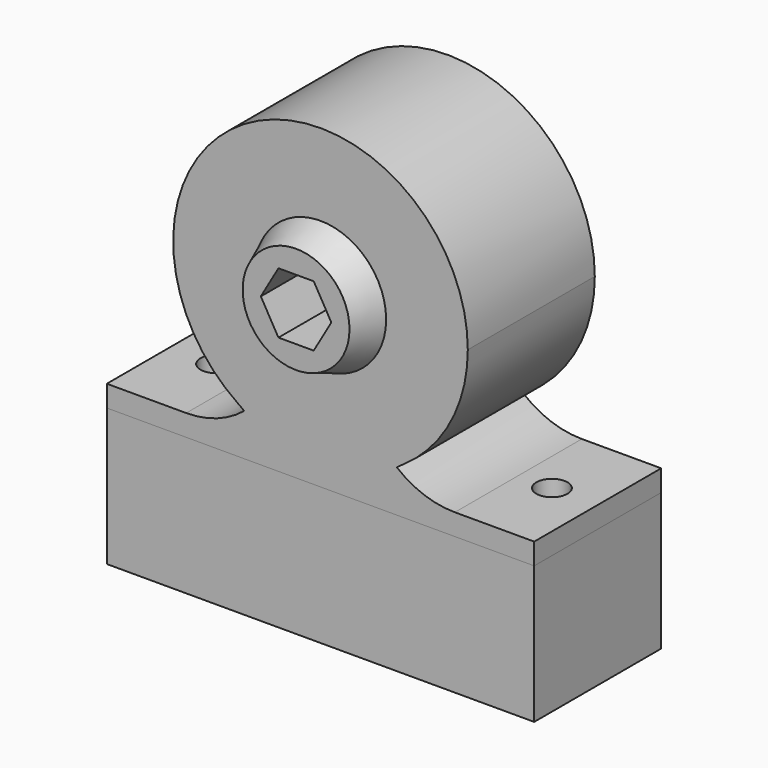
from build123d import *

# Parameters (mm, degrees)
F0_R         = 10.75
F1_DEPTH     = 26
F2_W         = 14
F2_H         = 26
F3_DEPTH     = 2
F4_T1_DEPTH  = 26
F4_T6_DEPTH  = 26
F4_T11_DEPTH = 26
F5_DEPTH     = 31
F6_SIZE2     = 5
F6_SIZE      = 2
F7_D         = 5.1054
F8_DEPTH     = 22.5


# Not quite as in the source:
# - a fillet or chamfer that OpenCascade refuses, or shapes differently, is made with other operations: its cross-section is extruded or revolved along the edge and cut away or added


with BuildPart() as f1:
    # F0 (on Front) → F1 (new body)
    with BuildSketch(Plane.XZ):
        with BuildLine():
            ThreePointArc((4.14e-08, -24.125), (17.0589511108, -17.0589510815), (24.125, 0))
            ThreePointArc((24.125, 0), (-17.0589511108, 17.0589510815), (4.14e-08, -24.125))
        make_face()
        Circle(F0_R, mode=Mode.SUBTRACT)
    extrude(amount=F1_DEPTH)



with BuildPart() as f1b:
    # F0 (on Front) → F1, piece 2 (new body)
    with BuildSketch(Plane.XZ):
        Polygon((35, -24.125), (4.14e-08, -24.125), (-35, -24.125), (-35, -27.625), (35, -27.625), align=None)
    extrude(amount=F1_DEPTH)


with BuildPart() as f1_1:
    add(f1.part)

    add(f1b.part)  # F3 merges F1b
    # F2 (on face) → F3 (join)
    with BuildSketch(Plane.XY.offset(-24.125)):
        with Locations((0, -13)):
            Rectangle(F2_W, F2_H)
    extrude(amount=F3_DEPTH)

    # F4: fillet of radius 15 on 4 edges, made by hand

    # F4_s2 → F4_t1 (join)
    with BuildSketch(Plane.XZ):
        with BuildLine():
            ThreePointArc((-22, -24.125), (-11.3933982822, -19.7316017178), (-7, -9.125))
            Line((-7, -9.125), (-7, -24.125))
            Line((-7, -24.125), (-22, -24.125))
        make_face()
        with BuildLine():
            ThreePointArc((22, -24.125), (11.3933982822, -19.7316017178), (7, -9.125))
            Line((7, -9.125), (7, -24.125))
            Line((7, -24.125), (22, -24.125))
        make_face()
    extrude(amount=F4_T1_DEPTH)


with BuildPart() as f4_tool4:
    # F4_s5 → F4_t6 (new body)
    with BuildSketch(Plane.XZ.offset(26)):
        with BuildLine():
            ThreePointArc((7, -32.3537575098), (8.7425950525, -25.3365490863), (13.5654952077, -19.9497610204))
            ThreePointArc((13.5654952077, -19.9497610204), (10.4017148166, -21.7674057681), (7, -23.0871311557))
            Line((7, -23.0871311557), (7, -32.3537575098))
        make_face()
    extrude(amount=-F4_T6_DEPTH)

    split(bisect_by=Plane.XY.offset(-27.625), keep=Keep.TOP)


with BuildPart() as f1_2:
    add(f1_1.part)

    # F4_t3: union F4_tool4
    add(f4_tool4.part)


with BuildPart() as f4_tool9:
    # F4_s10 → F4_t11 (new body)
    with BuildSketch(Plane.XZ.offset(26)):
        with BuildLine():
            ThreePointArc((-13.5654952077, -19.9497610204), (-8.7425950525, -25.3365490863), (-7, -32.3537575098))
            Line((-7, -32.3537575098), (-7, -23.0871311557))
            ThreePointArc((-7, -23.0871311557), (-10.4017148166, -21.7674057681), (-13.5654952077, -19.9497610204))
        make_face()
    extrude(amount=-F4_T11_DEPTH)

    split(bisect_by=Plane.XY.offset(-27.625), keep=Keep.TOP)


with BuildPart() as f1_3:
    add(f1_2.part)

    # F4_t8: union F4_tool9
    add(f4_tool9.part)

    # F7 (through all)
    with Locations(Plane.XY.offset(-24.125)):
        with Locations((-27.5, -13), (27.5, -13)):
            Hole(F7_D / 2)


with BuildPart() as f5:
    # F0 (on Front) → F5 (new body)
    with BuildSketch(Plane.XZ):
        Circle(F0_R)
        Polygon((-5.7735026919, 0), (-2.8867513459, 5), (2.8867513459, 5), (5.7735026919, 0), (2.8867513459, -5), (-2.8867513459, -5), align=None, mode=Mode.SUBTRACT)
    extrude(amount=F5_DEPTH)

    # F6
    f6_edges = [f5.edges().sort_by_distance(p)[0] for p in [
        (-10.75, -31, 0),
    ]]
    f6_side = f5.faces().sort_by_distance((-10.445944, -31, 0))[0]
    chamfer(f6_edges, length=F6_SIZE, length2=F6_SIZE2, reference=f6_side)


with BuildPart() as f8:
    # F8 (new): a face of the model
    f8_faces = [f1_3.part.faces().sort_by_distance(p)[0] for p in [
        (0, -13, -27.625),
    ]]
    extrude(f8_faces, amount=F8_DEPTH)


solid = Compound([f1_3.part, f5.part, f8.part])
